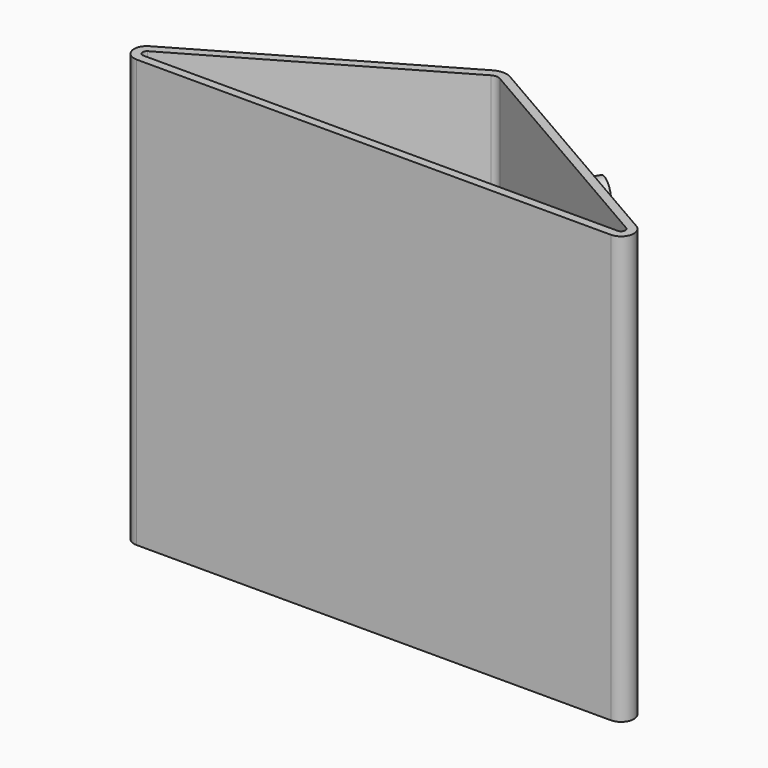
from build123d import *

# Parameters (mm, degrees)
F1_DEPTH = 150
F2_R     = 5
F3_DEPTH = 20


# Not quite as in the source:
# - a pattern or mirror of a feature is missing from the dataset's text; its kind, count and spacing are read off the source's solid


with BuildPart() as f1:
    # F0 (on Top) → F1 (new body)
    with BuildSketch(Plane.XY):
        with BuildLine():
            Line((-83.2057713659, 0), (0, 0))
            Line((0, 0), (83.2057713659, 0))
            ThreePointArc((83.2057713659, 0), (87.5524375842, 3.335314297), (85.4557713659, 8.397114317))
            Line((85.4557713659, 8.397114317), (3, 56.0029761114))
            ThreePointArc((3, 56.0029761114), (0, 56.8068236887), (-3, 56.0029761114))
            Line((-3, 56.0029761114), (-85.4557713659, 8.397114317))
            ThreePointArc((-85.4557713659, 8.397114317), (-87.5524375842, 3.335314297), (-83.2057713659, 0))
        make_face()
        with BuildLine():
            Line((83.2057713659, 3), (0, 3))
            Line((0, 3), (-83.2057713659, 3))
            ThreePointArc((-83.2057713659, 3), (-84.6546601054, 4.1117714323), (-83.9557713659, 5.7990381057))
            Line((-83.9557713659, 5.7990381057), (-1.5, 53.4048999))
            ThreePointArc((-1.5, 53.4048999), (0, 53.8068236887), (1.5, 53.4048999))
            Line((1.5, 53.4048999), (83.9557713659, 5.7990381057))
            ThreePointArc((83.9557713659, 5.7990381057), (84.6546601054, 4.1117714323), (83.2057713659, 3))
        make_face(mode=Mode.SUBTRACT)
    extrude(amount=F1_DEPTH)

    # F2 (on face) → F3 (join)
    with BuildSketch(Plane(origin=(-25, 43.3012701892, 0), x_dir=(-0.8660254038, -0.5, 0), z_dir=(-0.5, 0.8660254038, 0))):
        with Locations((-5.4034118443, 30)):
            Circle(F2_R)
        with Locations((-5.4034118443, 120)):
            Circle(F2_R)
    f3 = extrude(amount=F3_DEPTH)

    # F3_copies: F3 across plane
    add(f3.mirror(Plane(origin=(0, 0, 0), x_dir=(0, 0, 1), z_dir=(1, 0, 0))))


solid = f1.part
